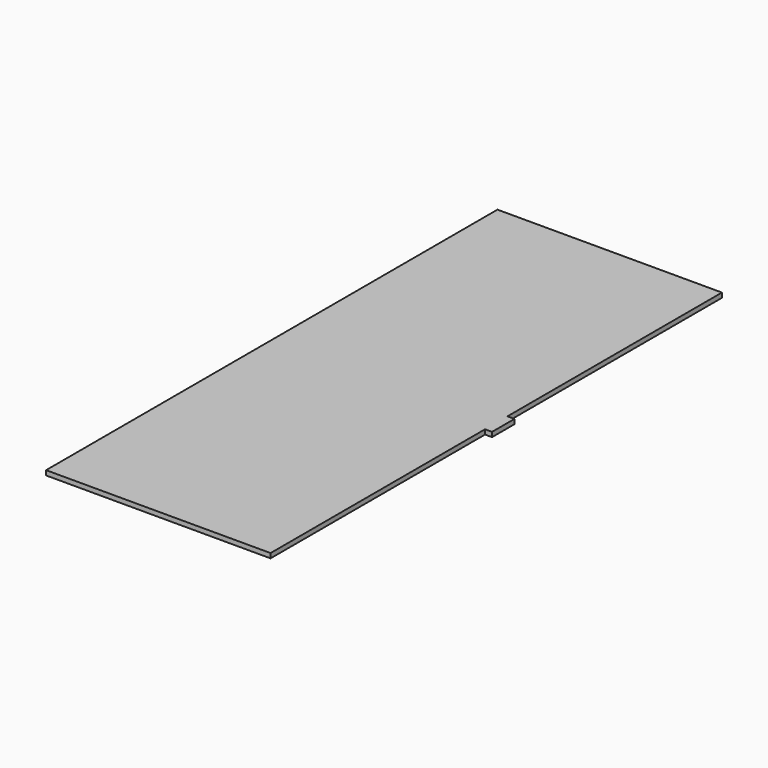
from build123d import *

# Parameters (mm, degrees)
F0_W     = 117.65
F0_H     = 2
F0_W_2   = 12
F1_DEPTH = 96
F2_DEPTH = 3
F3_DEPTH = 2
F4_DEPTH = 2
F5_DEPTH = 1
F6_DEPTH = 1


with BuildPart() as f1:
    # F0 (on Right) → F1 (new body)
    with BuildSketch(Plane.YZ):
        with Locations((244.2264966011, 75.535411799)):
            Rectangle(F0_W, F0_H)
        with Locations((179.4014966011, 75.535411799)):
            Rectangle(F0_W_2, F0_H)
        with Locations((114.5764966011, 75.535411799)):
            Rectangle(F0_W, F0_H)
    extrude(amount=-F1_DEPTH)

    # F0 (on Right) → F2 (join)
    with BuildSketch(Plane.YZ):
        with Locations((179.4014966011, 75.535411799)):
            Rectangle(F0_W_2, F0_H)
    extrude(amount=F2_DEPTH)

    # F3 (cut): a face of the model
    f3_faces = [f1.faces().sort_by_distance(p)[0] for p in [
        (-48, 55.7514966011, 75.535411799),
    ]]
    extrude(f3_faces, amount=-F3_DEPTH, mode=Mode.SUBTRACT)

    # F4 (cut): a face of the model
    f4_faces = [f1.faces().sort_by_distance(p)[0] for p in [
        (-48, 303.0514966011, 75.535411799),
    ]]
    extrude(f4_faces, amount=-F4_DEPTH, mode=Mode.SUBTRACT)

    # F5 (cut): a face of the model
    f5_faces = [f1.faces().sort_by_distance(p)[0] for p in [
        (-48, 57.7514966011, 75.535411799),
    ]]
    extrude(f5_faces, amount=-F5_DEPTH, mode=Mode.SUBTRACT)

    # F6 (cut): a face of the model
    f6_faces = [f1.faces().sort_by_distance(p)[0] for p in [
        (-48, 301.0514966011, 75.535411799),
    ]]
    extrude(f6_faces, amount=-F6_DEPTH, mode=Mode.SUBTRACT)


solid = f1.part
